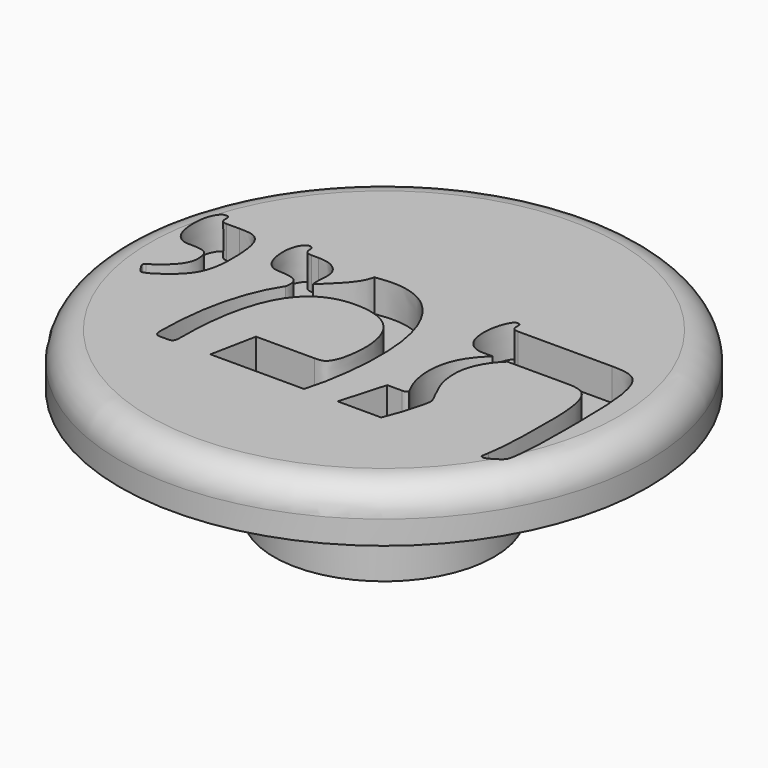
from build123d import *

# Parameters (mm, degrees)
F0_R         = 9
F1_DEPTH     = 1.8
F2_R         = 3.75
F3_DEPTH     = 3.8
F4_TEXT_SIZE = 11.1022093477
F5_DEPTH     = 1.1


# Not quite as in the source:
# - a fillet or chamfer that OpenCascade refuses, or shapes differently, is made with other operations: its cross-section is extruded or revolved along the edge and cut away or added
# - Text() gives the source's letters only with a copy of the font that has no kerning and outlines rounded to 1/6400 em; it was checked with that copy


with BuildPart() as f1:
    # F0 (on Top) → F1 (new body)
    with BuildSketch(Plane.XY):
        Circle(F0_R)
    extrude(amount=-F1_DEPTH)

    # F2 (on face) → F3 (join)
    with BuildSketch(Plane(origin=(0, 0, -1.8), x_dir=(1, 0, 0), z_dir=(0, 0, -1))):
        Circle(F2_R)
    extrude(amount=F3_DEPTH)

    # F4 (on face) → F5 (cut)
    with BuildSketch(Plane.XY):
        with Locations((-8.0638468989, -3.9967953652)):
            Text('ימת', F4_TEXT_SIZE, font='Tinos', font_style=FontStyle.BOLD, text_align=(TextAlign.LEFT, TextAlign.BOTTOM))
    extrude(amount=-F5_DEPTH, mode=Mode.SUBTRACT)

    # F6: fillet of radius 1 on 1 edges, made by hand

    # F6_s1 → F6_t2 (revolve, cut)
    with BuildSketch(Plane.XZ):
        with BuildLine():
            ThreePointArc((9, -1), (8.7071067812, -0.2928932188), (8, 0))
            Line((8, 0), (9, 0))
            Line((9, 0), (9, -1))
        make_face()
    revolve(axis=Axis((0, 0, 0), (0, 0, 1)), mode=Mode.SUBTRACT)


solid = f1.part
